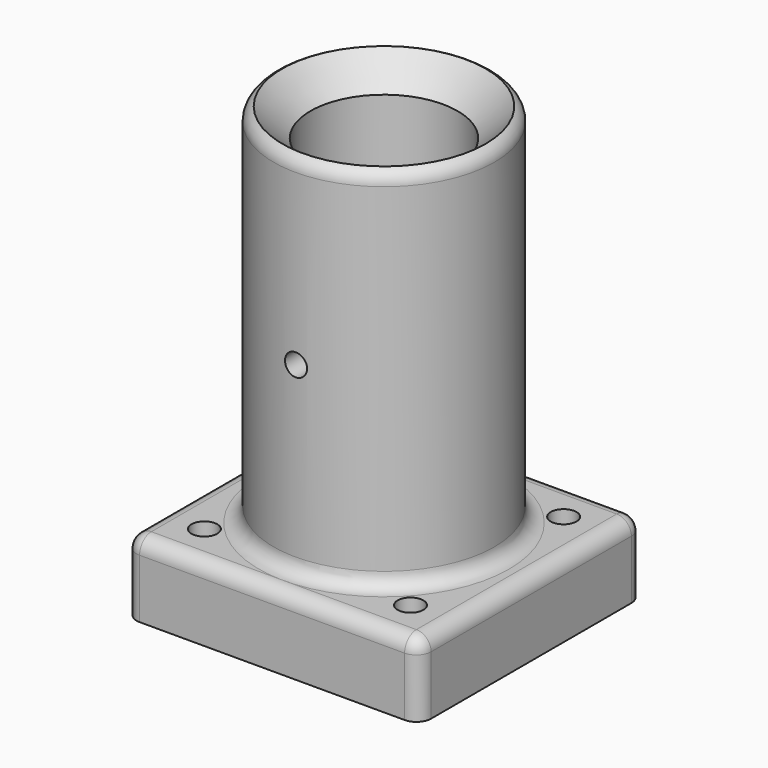
from build123d import *

# Parameters (mm, degrees)
F0_W     = 40
F0_H     = 38
F0_R     = 10
F1_DEPTH = 10
F4_D     = 3.5
F2_R     = 15
F2_R_2   = 10
F5_DEPTH = 50
F6_R     = 1.5
F7_DEPTH = 25
F8_R     = 1.99999


# Not quite as in the source:
# - a fillet or chamfer that OpenCascade refuses, or shapes differently, is made with other operations: its cross-section is extruded or revolved along the edge and cut away or added
# - a fillet or chamfer is up to 0.001 mm smaller than in the source, because OpenCascade refuses the exact size


with BuildPart() as f1:
    # F0 (on Top) → F1 (new body)
    with BuildSketch(Plane.XY):
        Rectangle(F0_W, F0_H)
        Circle(F0_R, mode=Mode.SUBTRACT)
    extrude(amount=F1_DEPTH)

    # F4 (through all)
    with Locations(Plane.XY.offset(10)):
        with Locations((-14, 13), (-14, -13), (14, -13), (14, 13)):
            Hole(F4_D / 2)

    # F2 (on face) → F5 (join)
    with BuildSketch(Plane.XY.offset(10)):
        Circle(F2_R)
        Circle(F2_R_2, mode=Mode.SUBTRACT)
    extrude(amount=F5_DEPTH)

    # F6 (on Front) → F7 (cut)
    with BuildSketch(Plane.XZ):
        with Locations((0, 35)):
            Circle(F6_R)
    extrude(amount=F7_DEPTH, mode=Mode.SUBTRACT)

    # F8 (radius 2 in the source; OpenCascade refuses exactly that, so slightly less here)
    f8_edges = [f1.edges().sort_by_distance(p)[0] for p in [
        (-15, 0, 10),
        (20, 0, 10),
        (0, -19, 10),
        (-20, 0, 10),
        (0, 19, 10),
        (20, 19, 5),
        (-20, -19, 5),
        (20, -19, 5),
        (-15, 0, 60),
        (-20, 19, 5),
    ]]
    fillet(f8_edges, radius=F8_R)

    # F9: chamfer of 4 on 1 edges, made by hand

    # F9_s1 → F9_t2 (revolve, cut)
    with BuildSketch(Plane.XZ):
        Polygon((10, 56), (14, 60), (10, 60), align=None)
    revolve(axis=Axis((0, 0, 60), (0, 0, 1)), mode=Mode.SUBTRACT)


solid = f1.part
